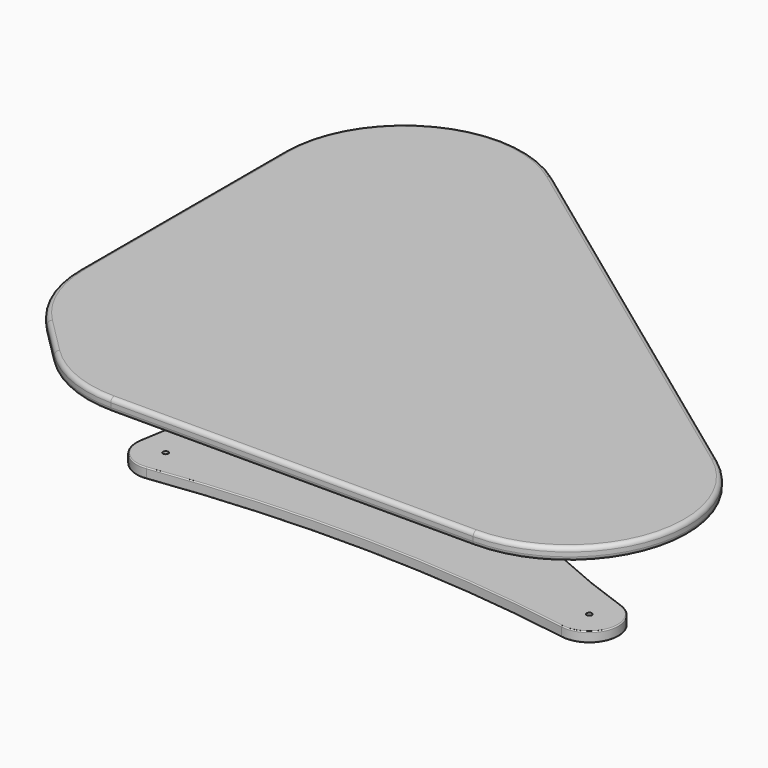
from build123d import *

# Parameters (mm, degrees)
F0_R     = 5
F1_DEPTH = 24
F2_START = -15
F2_DEPTH = 9.001
F3_R     = 8
F4_START = -204
F4_DEPTH = 19
F5_R     = 2


# Not quite as in the source:
# - a feature names something its author has since deleted; it is built from what else it names


with BuildPart() as f1:
    # F0 (on Top) → F1 (new body)
    with BuildSketch(Plane.XY):
        with BuildLine():
            ThreePointArc((358.0568243162, 956.4411240675), (123.2964736873, 975.7022489549), (0, 775))
            Line((0, 775), (0, 293.1980515339))
            ThreePointArc((0, 293.1980515339), (17.127105185, 207.0942792518), (65.900974233, 134.099025767))
            Line((65.900974233, 134.099025767), (134.099025767, 65.900974233))
            ThreePointArc((134.099025767, 65.900974233), (207.0942792518, 17.127105185), (293.1980515339, 0))
            Line((293.1980515339, 0), (975, 0))
            ThreePointArc((975, 0), (1188.8331743617, 154.9973318908), (1108.0568243162, 406.4411240675))
            Line((1108.0568243162, 406.4411240675), (358.0568243162, 956.4411240675))
        make_face()
        with BuildLine():
            ThreePointArc((146.9597475721, 810.0268739765), (176.7826648554, 873.8548809714), (244.9290040162, 855.9803926927))
            ThreePointArc((244.9290040162, 855.9803926927), (598.2074073313, 495.1712029306), (1045.0353645703, 259.9400861638))
            ThreePointArc((1045.0353645703, 259.9400861638), (1080.5893950333, 194.3946501102), (1018.1368916862, 153.651821351))
            ThreePointArc((1018.1368916862, 153.651821351), (623.3674740325, 189.6950371654), (227.6818379424, 165.7183002563))
            ThreePointArc((227.6818379424, 165.7183002563), (180.2577174949, 182.4065295721), (166.2142552173, 230.6799732568))
            ThreePointArc((166.2142552173, 230.6799732568), (189.282478165, 521.4400528998), (146.9597475721, 810.0268739765))
        make_face(mode=Mode.SUBTRACT)
        with BuildLine():
            ThreePointArc((1045.0353645703, 259.9400861638), (598.2074073313, 495.1712029306), (244.9290040162, 855.9803926927))
            ThreePointArc((244.9290040162, 855.9803926927), (176.7826648554, 873.8548809714), (146.9597475721, 810.0268739765))
            ThreePointArc((146.9597475721, 810.0268739765), (189.282478165, 521.4400528998), (166.2142552173, 230.6799732568))
            ThreePointArc((166.2142552173, 230.6799732568), (180.2577174949, 182.4065295721), (227.6818379424, 165.7183002563))
            ThreePointArc((227.6818379424, 165.7183002563), (623.3674740325, 189.6950371654), (1018.1368916862, 153.651821351))
            ThreePointArc((1018.1368916862, 153.651821351), (1080.5893950333, 194.3946501102), (1045.0353645703, 259.9400861638))
        make_face()
        with Locations((220.2081528017, 220.2081528017)):
            Circle(F0_R, mode=Mode.SUBTRACT)
        with Locations((1027.2703072802, 207.8881626692)):
            Circle(F0_R, mode=Mode.SUBTRACT)
        with Locations((200.1392074826, 824.0605849477)):
            Circle(F0_R, mode=Mode.SUBTRACT)
        with Locations((220.2081528017, 220.2081528017)):
            Circle(F0_R)
        with Locations((200.1392074826, 824.0605849477)):
            Circle(F0_R)
        with Locations((1027.2703072802, 207.8881626692)):
            Circle(F0_R)
    extrude(amount=-F1_DEPTH)

    # F0 (on Top) → F2 (cut)
    with BuildSketch(Plane.XY.offset(F2_START)):
        with Locations((1027.2703072802, 207.8881626692)):
            Circle(F0_R)
        with Locations((220.2081528017, 220.2081528017)):
            Circle(F0_R)
        with Locations((200.1392074826, 824.0605849477)):
            Circle(F0_R)
    extrude(amount=-F2_DEPTH, mode=Mode.SUBTRACT)

    # F3
    f3_edges = [f1.edges().sort_by_distance(p)[0] for p in [
        (100, 100, 0),
        (634.099026, 0, -24),
    ]]
    fillet(f3_edges, radius=F3_R)


with BuildPart() as f4:
    # F0 (on Top) → F4 (new body)
    with BuildSketch(Plane.XY.offset(F4_START)):
        with BuildLine():
            ThreePointArc((1045.0353645703, 259.9400861638), (598.2074073313, 495.1712029306), (244.9290040162, 855.9803926927))
            ThreePointArc((244.9290040162, 855.9803926927), (176.7826648554, 873.8548809714), (146.9597475721, 810.0268739765))
            ThreePointArc((146.9597475721, 810.0268739765), (189.282478165, 521.4400528998), (166.2142552173, 230.6799732568))
            ThreePointArc((166.2142552173, 230.6799732568), (180.2577174949, 182.4065295721), (227.6818379424, 165.7183002563))
            ThreePointArc((227.6818379424, 165.7183002563), (623.3674740325, 189.6950371654), (1018.1368916862, 153.651821351))
            ThreePointArc((1018.1368916862, 153.651821351), (1080.5893950333, 194.3946501102), (1045.0353645703, 259.9400861638))
        make_face()
        with Locations((220.2081528017, 220.2081528017)):
            Circle(F0_R, mode=Mode.SUBTRACT)
        with Locations((1027.2703072802, 207.8881626692)):
            Circle(F0_R, mode=Mode.SUBTRACT)
        with Locations((200.1392074826, 824.0605849477)):
            Circle(F0_R, mode=Mode.SUBTRACT)
    extrude(amount=-F4_DEPTH)

    # F5
    f5_edges = [f4.edges().sort_by_distance(p)[0] for p in [
        (623.367474, 189.695037, -204),
        (623.367474, 189.695037, -223),
    ]]
    fillet(f5_edges, radius=F5_R)


solid = Compound([f1.part, f4.part])
